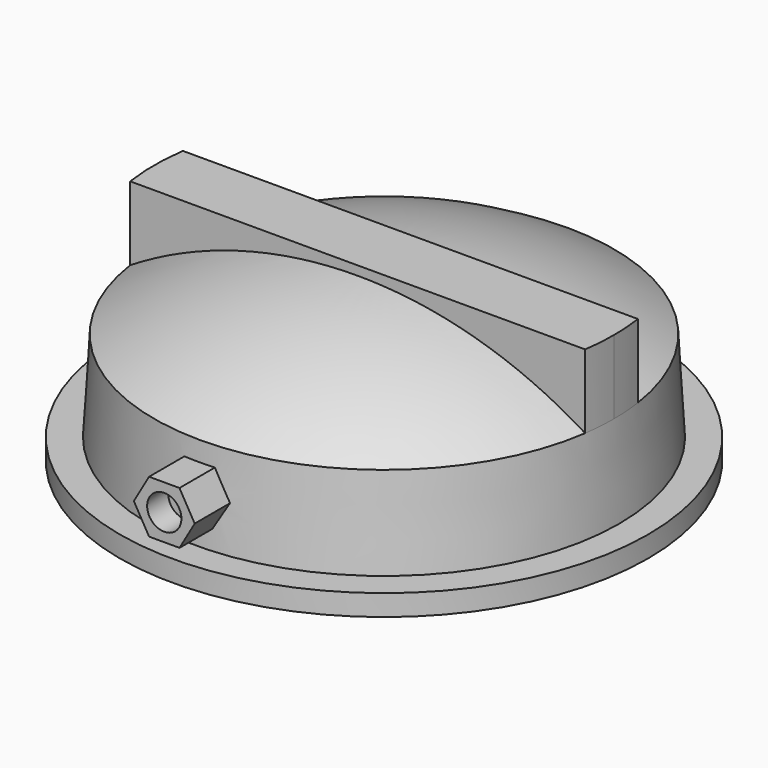
from build123d import *

# Parameters (mm, degrees)
F0_R      = 43.6
F2_R      = 44.6
F4_R      = 50.1
F4_R_2    = 44.6
F5_DEPTH  = 4
F13_DEPTH = 8.5
F14_R     = 3.25
F15_DEPTH = 5


with BuildPart() as f3:
    # F0 (on Top) → F3 section 0
    with BuildSketch(Plane.XY):
        Circle(F0_R)
    # F2 (on offset) → F3 section 1
    with BuildSketch(Plane.XY.offset(-17.2)):
        Circle(F2_R)
    loft()

    # F4 (on face) → F5 (join)
    with BuildSketch(Plane(origin=(0, 0, -17.2), x_dir=(1, 0, 0), z_dir=(0, 0, -1))):
        Circle(F4_R)
        Circle(F4_R_2, mode=Mode.SUBTRACT)
        Circle(F4_R_2)
    extrude(amount=F5_DEPTH)

    # F6 (on Front) → F7 (revolve)
    with BuildSketch(Plane.XZ):
        with BuildLine():
            Line((-43.6, 0), (0, 0))
            Line((0, 0), (0, 12.5))
            ThreePointArc((0, 12.5), (-22.6782384677, 9.3132957755), (-43.6, 0))
        make_face()
    revolve(axis=Axis((0, 0, 11.7095857859), (0, 0, 1)))

    # F9 (on offset) → F10 (join, up to the next surface of F3)
    with BuildSketch(Plane.XY.offset(14)):
        with BuildLine():
            ThreePointArc((43.6, 0), (43.4872818741, 3.1330999347), (43.1497103119, 6.25))
            Line((43.1497103119, 6.25), (-43.1497103119, 6.25))
            ThreePointArc((-43.1497103119, 6.25), (-43.6, 0), (-43.1497103119, -6.25))
            Line((-43.1497103119, -6.25), (43.1497103119, -6.25))
            ThreePointArc((43.1497103119, -6.25), (43.4872818741, -3.1330999347), (43.6, 0))
        make_face()
    extrude(until=Until.NEXT, dir=(0, 0, -1))

    # F12 (on offset) → F13 (join)
    with BuildSketch(Plane.XZ.offset(43.6)):
        Polygon((2.8867513459, -13.6), (5.7735026919, -8.6), (2.8867513459, -3.6), (-2.8867513459, -3.6), (-5.7735026919, -8.6), (-2.8867513459, -13.6), align=None)
    extrude(amount=F13_DEPTH)

    # F14 (on face) → F15 (cut)
    with BuildSketch(Plane.XZ.offset(52.1)):
        with Locations((0, -8.6)):
            Circle(F14_R)
    extrude(amount=-F15_DEPTH, mode=Mode.SUBTRACT)


solid = f3.part
